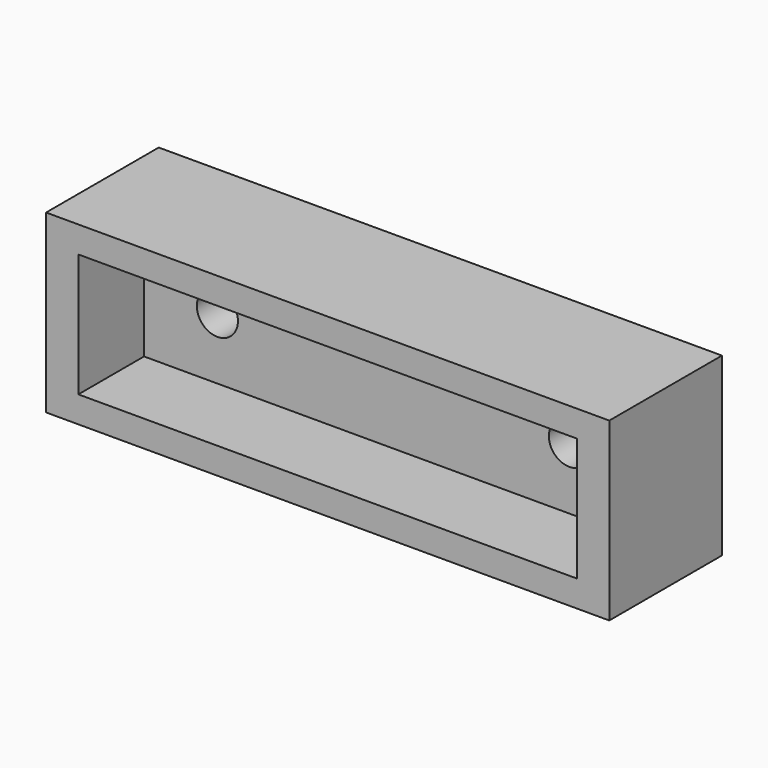
from build123d import *

# Parameters (mm, degrees)
F0_W     = 48
F0_H     = 15
F1_DEPTH = 12
F2_W     = 42.5
F2_H     = 10.5
F3_DEPTH = 7
F4_R     = 1.75
F5_DEPTH = 5


# Not quite as in the source:
# - a pattern or mirror of a feature is missing from the dataset's text; its kind, count and spacing are read off the source's solid


with BuildPart() as f1:
    # F0 (on Front) → F1 (new body)
    with BuildSketch(Plane.XZ):
        Rectangle(F0_W, F0_H)
    extrude(amount=F1_DEPTH)

    # F2 (on face) → F3 (cut)
    with BuildSketch(Plane.XZ.offset(12)):
        Rectangle(F2_W, F2_H)
    extrude(amount=-F3_DEPTH, mode=Mode.SUBTRACT)

    # F4 (on face) → F5 (cut, through all)
    with BuildSketch(Plane.XZ.offset(5)):
        with Locations((-15, 0)):
            Circle(F4_R)
    f5 = extrude(amount=-F5_DEPTH, mode=Mode.SUBTRACT)

    # F5_copies: F5 across plane
    add(f5.mirror(Plane(origin=(0, 0, 0), x_dir=(0, 0, 1), z_dir=(1, 0, 0))), mode=Mode.SUBTRACT)


solid = f1.part
